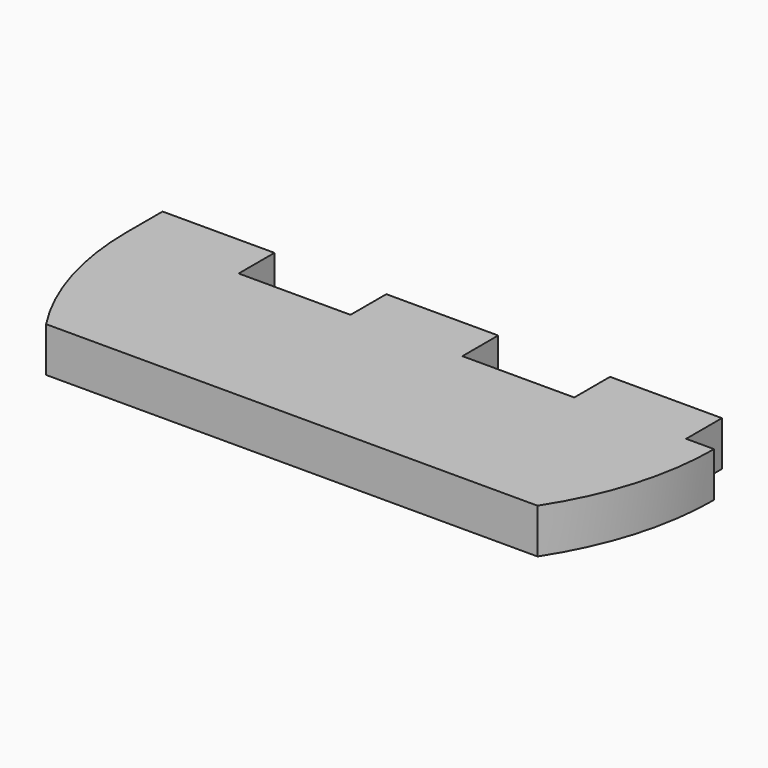
from build123d import *

# Parameters (mm, degrees)
F1_DEPTH = 1.6


# Not quite as in the source:
# - a feature names something its author has since deleted; it is built from what else it names


with BuildPart() as f1:
    # F0 (on Top) → F1 (new body, symmetric)
    with BuildSketch(Plane.XY):
        with BuildLine():
            Line((-21, 3.2), (-21, 0))
            ThreePointArc((-21, 0), (-20.1245739235, -6.0001270317), (-17.5712833908, -11.5))
            Line((-17.5712833908, -11.5), (0, -11.5))
            Line((0, -11.5), (17.5712833908, -11.5))
            ThreePointArc((17.5712833908, -11.5), (20.1245739235, -6.0001270317), (21, 0))
            Line((21, 0), (19, 0))
            Line((19, 0), (19, 3.2))
            Line((19, 3.2), (11, 3.2))
            Line((11, 3.2), (11, 0))
            Line((11, 0), (3, 0))
            Line((3, 0), (3, 3.2))
            Line((3, 3.2), (-5, 3.2))
            Line((-5, 3.2), (-5, 0))
            Line((-5, 0), (-13, 0))
            Line((-13, 0), (-13, 3.2))
            Line((-13, 3.2), (-21, 3.2))
        make_face()
    extrude(amount=F1_DEPTH, both=True)


solid = f1.part
